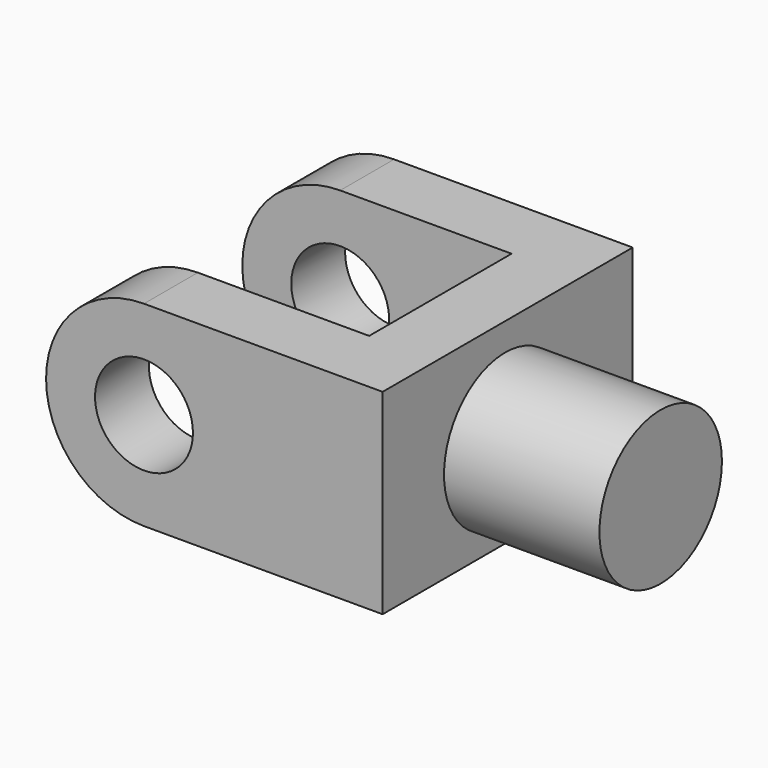
from build123d import *

# Parameters (mm, degrees)
F1_DEPTH  = 32
F2_R      = 16
F3_R      = 15.99999
F4_R      = 16
F5_R      = 15.99999
F6_R      = 8
F7_DEPTH  = 25.4
F8_R      = 8
F9_DEPTH  = 25.4
F10_R     = 12.5095984865
F11_DEPTH = 25.4


# Not quite as in the source:
# - a fillet or chamfer is up to 0.001 mm smaller than in the source, because OpenCascade refuses the exact size


with BuildPart() as f1:
    # F0 (on Top) → F1 (new body)
    with BuildSketch(Plane.XY):
        Polygon((55, -31.1075148418), (55, 19.9773363869), (0, 19.9773363869), (0, 8.9773363869), (44, 8.9773363869), (44, -20.1075148418), (0, -20.1075148418), (0, -31.1075148418), align=None)
    extrude(amount=F1_DEPTH)

    # F2
    f2_edges = [f1.edges().sort_by_distance(p)[0] for p in [
        (0, -25.607515, 32),
    ]]
    fillet(f2_edges, radius=F2_R)

    # F3 (radius 16 in the source; OpenCascade refuses exactly that, so slightly less here)
    f3_edges = [f1.edges().sort_by_distance(p)[0] for p in [
        (0, -25.607515, 0),
    ]]
    fillet(f3_edges, radius=F3_R)

    # F4
    f4_edges = [f1.edges().sort_by_distance(p)[0] for p in [
        (0, 14.477336, 32),
    ]]
    fillet(f4_edges, radius=F4_R)

    # F5 (radius 16 in the source; OpenCascade refuses exactly that, so slightly less here)
    f5_edges = [f1.edges().sort_by_distance(p)[0] for p in [
        (0, 14.477336, 0),
    ]]
    fillet(f5_edges, radius=F5_R)

    # F6 (on face) → F7 (cut)
    with BuildSketch(Plane(origin=(0, 19.9773363869, 0), x_dir=(-1, 0, 0), z_dir=(0, 1, 0))):
        with Locations((-16, 16)):
            Circle(F6_R)
    extrude(amount=-F7_DEPTH, mode=Mode.SUBTRACT)

    # F8 (on face) → F9 (cut)
    with BuildSketch(Plane.XZ.offset(31.1075148418)):
        with Locations((16, 16)):
            Circle(F8_R)
    extrude(amount=-F9_DEPTH, mode=Mode.SUBTRACT)

    # F10 (on face) → F11 (join)
    with BuildSketch(Plane.YZ.offset(55)):
        with Locations((-6.0587972403, 14.9832107127)):
            Circle(F10_R)
    extrude(amount=F11_DEPTH)


solid = f1.part
